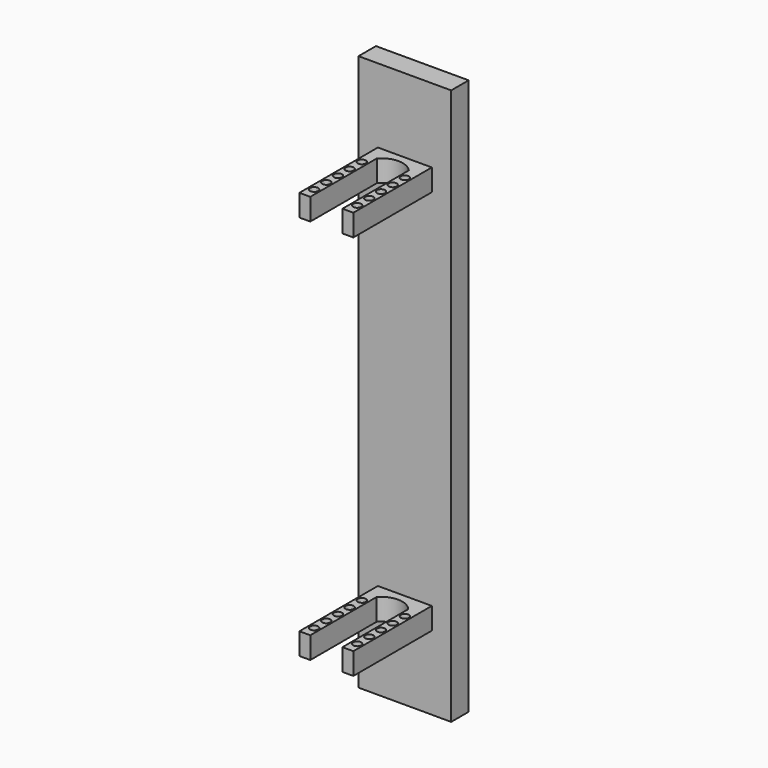
from build123d import *

# Parameters (mm, degrees)
F0_W      = 125.73
F0_H      = 172.72
F0_H_2    = 848.614
F0_H_3    = 172.466
F1_DEPTH  = 50.8
F0_H_4    = 50.8
F2_DEPTH  = 279.4
F3_W      = 74.93
F3_H      = 4.6193234962
F4_DEPTH  = 154.94
F5_W      = 74.93
F5_H      = 11.4905911902
F6_DEPTH  = 111.76
F7_R      = 9.525
F9_DEPTH  = 53.34
F10_R     = 9.525
F11_DEPTH = 53.34
F12_R     = 9.525
F13_DEPTH = 53.34


# Not quite as in the source:
# - a feature names something its author has since deleted; it is built from what else it names


with BuildPart() as f1:
    # F0 (on Front) → F1 (new body)
    with BuildSketch(Plane.XZ):
        with Locations((-107.95, 86.36)):
            Rectangle(F0_W, F0_H)
        with Locations((-107.95, -475.107)):
            Rectangle(F0_W, F0_H_2)
        with Locations((-107.95, -1036.447)):
            Rectangle(F0_W, F0_H_3)
        Polygon((-170.815, 0), (-170.815, 172.72), (-215.9, 172.72), (-215.9, -1122.68), (-170.815, -1122.68), (-170.815, -950.214), (-170.815, -899.414), (-170.815, -50.8), align=None)
        Polygon((0, 172.72), (-45.085, 172.72), (-45.085, 0), (-45.085, -50.8), (-45.085, -899.414), (-45.085, -950.214), (-45.085, -1122.68), (-45.085, -1122.7624416351), (0, -1122.7624416351), align=None)
    extrude(amount=F1_DEPTH)


with BuildPart() as f2:
    # F0 (on Front) → F2 (new body)
    with BuildSketch(Plane.XZ):
        with Locations((-107.95, -25.4)):
            Rectangle(F0_W, F0_H_4)
    extrude(amount=F2_DEPTH)

    # F5 (on face) → F6 (cut)
    with BuildSketch(Plane.XY):
        with Locations((-107.95, -285.1452955951)):
            Rectangle(F5_W, F5_H)
        with BuildLine():
            Line((-145.415, -85.4969564537), (-145.415, -279.4))
            Line((-145.415, -279.4), (-70.485, -279.4))
            Line((-70.485, -279.4), (-70.485, -86.1544632))
            ThreePointArc((-70.485, -86.1544632), (-107.803229226, -69.0995938432), (-145.415, -85.4969564537))
        make_face()
    extrude(amount=-F6_DEPTH, mode=Mode.SUBTRACT)

    # F7 (on face) → F9 (cut)
    with BuildSketch(Plane.XY):
        with Locations((-57.785, -113.3856)):
            Circle(F7_R)
        with Locations((-57.785, -148.9456)):
            Circle(F7_R)
        with Locations((-57.785, -182.9181)):
            Circle(F7_R)
        with Locations((-57.785, -252.4506)):
            Circle(F7_R)
        with Locations((-57.785, -216.8906)):
            Circle(F7_R)
    extrude(amount=-F9_DEPTH, mode=Mode.SUBTRACT)

    # F10 (on face) → F11 (cut)
    with BuildSketch(Plane.XY):
        with Locations((-158.115, -113.3856)):
            Circle(F10_R)
        with Locations((-158.115, -148.9456)):
            Circle(F10_R)
        with Locations((-158.115, -182.9181)):
            Circle(F10_R)
        with Locations((-158.115, -216.8906)):
            Circle(F10_R)
        with Locations((-158.115, -252.4506)):
            Circle(F10_R)
    extrude(amount=-F11_DEPTH, mode=Mode.SUBTRACT)


with BuildPart() as f2b:
    # F0 (on Front) → F2, piece 2 (new body)
    with BuildSketch(Plane.XZ):
        with Locations((-107.95, -924.814)):
            Rectangle(F0_W, F0_H_4)
    extrude(amount=F2_DEPTH)

    # F3 (on face) → F4 (cut)
    with BuildSketch(Plane(origin=(0, 0, -950.214), x_dir=(1, 0, 0), z_dir=(0, 0, -1))):
        with Locations((-107.95, 281.7096617481)):
            Rectangle(F3_W, F3_H)
        with BuildLine():
            Line((-70.485, 87.6124339393), (-70.485, 279.4))
            Line((-70.485, 279.4), (-145.415, 279.4))
            Line((-145.415, 279.4), (-145.415, 86.1544632))
            ThreePointArc((-145.415, 86.1544632), (-107.617645147, 69.8026193953), (-70.485, 87.6124339393))
        make_face()
    extrude(amount=-F4_DEPTH, mode=Mode.SUBTRACT)

    # F12 (on face) → F13 (cut)
    with BuildSketch(Plane(origin=(0, 0, -950.214), x_dir=(1, 0, 0), z_dir=(0, 0, -1))):
        with Locations((-158.115, 113.3856)):
            Circle(F12_R)
        with Locations((-158.115, 148.9456)):
            Circle(F12_R)
        with Locations((-158.115, 182.9181)):
            Circle(F12_R)
        with Locations((-158.115, 216.8906)):
            Circle(F12_R)
        with Locations((-158.115, 252.4506)):
            Circle(F12_R)
        with Locations((-57.785, 113.3856)):
            Circle(F12_R)
        with Locations((-57.785, 148.9456)):
            Circle(F12_R)
        with Locations((-57.785, 182.9181)):
            Circle(F12_R)
        with Locations((-57.785, 216.8906)):
            Circle(F12_R)
        with Locations((-57.785, 252.4506)):
            Circle(F12_R)
    extrude(amount=-F13_DEPTH, mode=Mode.SUBTRACT)


solid = Compound([f1.part, f2.part, f2b.part])
